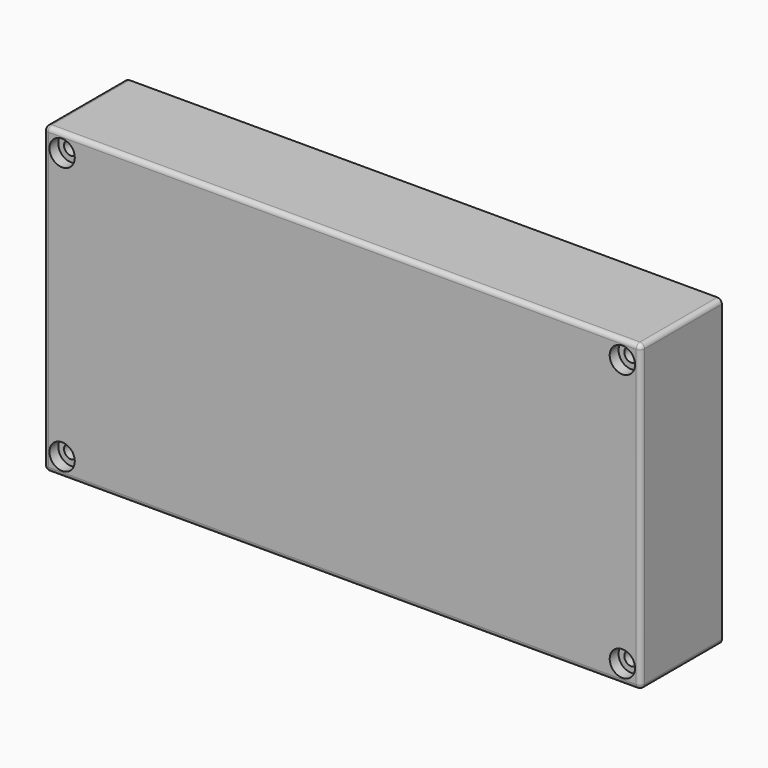
from build123d import *

# Parameters (mm, degrees)
F0_W           = 129.58
F0_H           = 66
F1_DEPTH       = 22
F3_D           = 3
F3_CBORE_D     = 5.5
F3_CBORE_DEPTH = 2.4
F4_T           = 2.54
F5_R           = 1


# Not quite as in the source:
# - a shell that OpenCascade refuses in one call is made with other operations: the cavity is built on its own and cut out


with BuildPart() as f1:
    # F0 (on Front) → F1 (new body)
    with BuildSketch(Plane.XZ):
        with Locations((64.79, 33)):
            Rectangle(F0_W, F0_H)
    extrude(amount=F1_DEPTH)

    # F3 (through all)
    with Locations(Plane.XZ.offset(22)):
        with Locations((4, 62), (4, 4), (125.58, 4), (125.58, 62)):
            CounterBoreHole(F3_D / 2, F3_CBORE_D / 2, F3_CBORE_DEPTH)

    # F4: shell of thickness 2.54, made by hand


with BuildPart() as f4_core1:
    # F4_t2: copy of F1
    add(f1.part)

    # the walls: a layer under each face that stays
    f4_faces = [f4_core1.faces().sort_by_distance(p)[0] for p in [
        (0, -11, 33),
        (64.79, -11, 66),
        (64.79, -11, 0),
        (64.79, -22, 33),
        (129.58, -11, 33),
        (2.5, -9.8, 4),
        (124.08, -9.8, 4),
        (2.5, -9.8, 62),
        (124.08, -9.8, 62),
        (1.25, -20.8, 4),
        (122.83, -20.8, 4),
        (1.25, -20.8, 62),
        (122.83, -20.8, 62),
        (2.1666666667, -19.6, 2.1666666667),
        (123.7466666667, -19.6, 2.1666666667),
        (2.1666666667, -19.6, 60.1666666667),
        (123.7466666667, -19.6, 60.1666666667),
    ]]
    thicken(f4_faces, amount=-F4_T, mode=Mode.SUBTRACT)

    # F4_s3 → F4_t4 (revolve, cut)
    with BuildSketch(Plane.XY.offset(4)):
        Polygon((6.7246, -19.6254), (9.29, -19.6), (9.29, -17.06), (6.75, -17.06), align=None)
    revolve(axis=Axis((4, -19.6, 4), (0, -1, 0)), mode=Mode.SUBTRACT)

    # F4_s5 → F4_t6 (revolve, cut)
    with BuildSketch(Plane.XY.offset(4)):
        Polygon((128.3046, -19.6254), (130.87, -19.6), (130.87, -17.06), (128.33, -17.06), align=None)
    revolve(axis=Axis((125.58, -19.6, 4), (0, -1, 0)), mode=Mode.SUBTRACT)

    # F4_s7 → F4_t8 (revolve, cut)
    with BuildSketch(Plane.XY.offset(62)):
        Polygon((6.7246, -19.6254), (9.29, -19.6), (9.29, -17.06), (6.75, -17.06), align=None)
    revolve(axis=Axis((4, -19.6, 62), (0, -1, 0)), mode=Mode.SUBTRACT)

    # F4_s9 → F4_t10 (revolve, cut)
    with BuildSketch(Plane.XY.offset(62)):
        Polygon((128.3046, -19.6254), (130.87, -19.6), (130.87, -17.06), (128.33, -17.06), align=None)
    revolve(axis=Axis((125.58, -19.6, 62), (0, -1, 0)), mode=Mode.SUBTRACT)


with BuildPart() as f1_1:
    add(f1.part)

    # what is left inside the walls is the cavity
    f4_cavity = [f4_core1.part.solids().sort_by_distance(p)[0] for p in [
        (64.79, -0.0254, 22.846667),
    ]]
    add(f4_cavity, mode=Mode.SUBTRACT)

    # F5
    f5_edges = [f1_1.edges().sort_by_distance(p)[0] for p in [
        (64.79, -22, 66),
        (0, -11, 66),
        (0, -11, 0),
        (129.58, -11, 66),
        (129.58, -11, 0),
        (64.79, -22, 0),
        (129.58, -22, 33),
        (0, -22, 33),
    ]]
    fillet(f5_edges, radius=F5_R)


solid = f1_1.part
